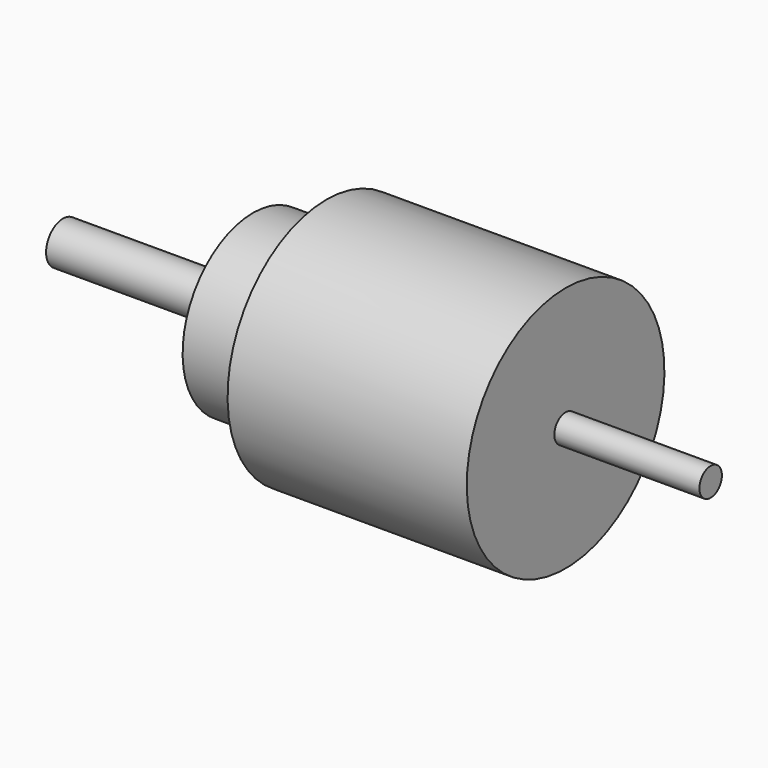
from build123d import *

# Parameters (mm, degrees)
F1_W = 20.61
F1_H = 2
F2_W = 59.51
F2_H = 2
F3_W = 27
F3_H = 3


with BuildPart() as f4:
    # F1 (on Front) → F4 (revolve)
    with BuildSketch(Plane.XZ):
        with Locations((10.305, 1)):
            Rectangle(F1_W, F1_H)
    revolve(axis=Axis((-25.4, 0, 0), (-1, 0, 0)))

    # F2 (on Front) → F5 (revolve)
    with BuildSketch(Plane.XZ):
        with Locations((-9.145, 1)):
            Rectangle(F2_W, F2_H)
    revolve(axis=Axis((-25.4, 0, 0), (-1, 0, 0)))


with BuildPart() as f4b:
    # F1 (on Front) → F4, piece 2 (revolve)
    with BuildSketch(Plane.XZ):
        Polygon((0, 17.55), (-33.9843811406, 17.55), (-36.9, 12.5), (-36.9, 2), (0, 2), align=None)
    revolve(axis=Axis((-25.4, 0, 0), (-1, 0, 0)))


with BuildPart() as f6:
    # F3 (on Front) → F6 (revolve)
    with BuildSketch(Plane.XZ):
        with Locations((-57.91, 1.5)):
            Rectangle(F3_W, F3_H)
        Polygon((-36.9, 12.5), (-44.41, 12.5), (-44.41, 3), (-44.41, 0), (-36.9, 0), align=None)
    revolve(axis=Axis((-25.4, 0, 0), (-1, 0, 0)))


solid = Compound([f4.part, f4b.part, f6.part])
